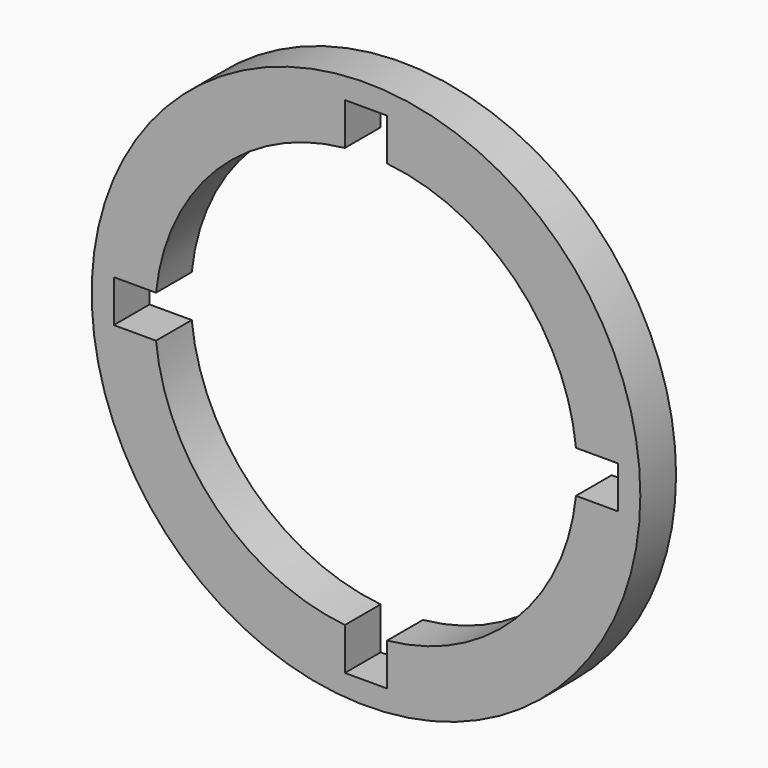
from build123d import *

# Parameters (mm, degrees)
F0_R     = 19.5
F1_DEPTH = 3.175


# Not quite as in the source:
# - a length typed as a fraction of an inch, garbled in the dataset ("3 / 203.2 mm" for 3/8 in), is restored


with BuildPart() as f1:
    # F0 (on Front) → F1 (new body)
    with BuildSketch(Plane.XZ):
        Circle(F0_R)
        with BuildLine():
            ThreePointArc((1.5, 14.9248115566), (10.6066017178, 10.6066017178), (14.9248115566, 1.5))
            Line((14.9248115566, 1.5), (17.9248115566, 1.5))
            Line((17.9248115566, 1.5), (17.9248115566, -1.5))
            Line((17.9248115566, -1.5), (14.9248115566, -1.5))
            ThreePointArc((14.9248115566, -1.5), (10.6066017178, -10.6066017178), (1.5, -14.9248115566))
            Line((1.5, -14.9248115566), (1.5, -17.9248115566))
            Line((1.5, -17.9248115566), (-1.5, -17.9248115566))
            Line((-1.5, -17.9248115566), (-1.5, -14.9248115566))
            ThreePointArc((-1.5, -14.9248115566), (-10.6066017178, -10.6066017178), (-14.9248115566, -1.5))
            Line((-14.9248115566, -1.5), (-17.9248115566, -1.5))
            Line((-17.9248115566, -1.5), (-17.9248115566, 1.5))
            Line((-17.9248115566, 1.5), (-14.9248115566, 1.5))
            ThreePointArc((-14.9248115566, 1.5), (-10.6066017178, 10.6066017178), (-1.5, 14.9248115566))
            Line((-1.5, 14.9248115566), (-1.5, 17.9248115566))
            Line((-1.5, 17.9248115566), (1.5, 17.9248115566))
            Line((1.5, 17.9248115566), (1.5, 14.9248115566))
        make_face(mode=Mode.SUBTRACT)
    extrude(amount=F1_DEPTH)


solid = f1.part
